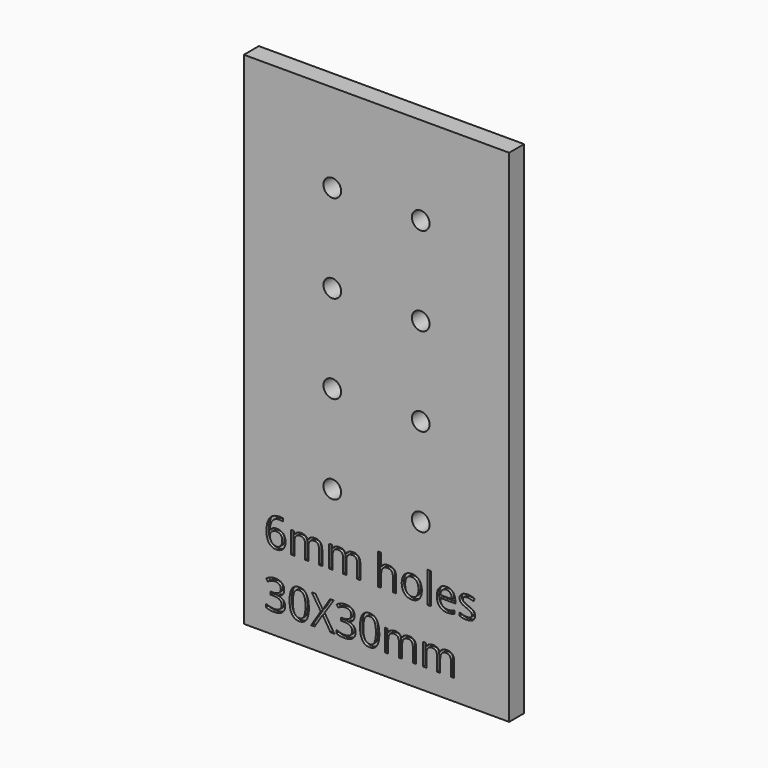
from build123d import *

# Parameters (mm, degrees)
F0_W         = 90
F0_H         = 170
F0_R         = 3
F1_DEPTH     = 6.35
F0_R_2       = 1.5
F3_TEXT_SIZE = 13.8888888889
F4_DEPTH     = 1


# Not quite as in the source:
# - Text() gives the source's letters only with a copy of the font that has no kerning and outlines rounded to 1/6400 em; it was checked with that copy


with BuildPart() as f1:
    # F0 (on Front) → F1 (new body)
    with BuildSketch(Plane.XZ):
        Rectangle(F0_W, F0_H)
        with Locations((-15, -35)):
            Circle(F0_R, mode=Mode.SUBTRACT)
        with Locations((-15, -5)):
            Circle(F0_R, mode=Mode.SUBTRACT)
        with Locations((15, -35)):
            Circle(F0_R, mode=Mode.SUBTRACT)
        with Locations((15, -5)):
            Circle(F0_R, mode=Mode.SUBTRACT)
        with Locations((-15, 25)):
            Circle(F0_R, mode=Mode.SUBTRACT)
        with Locations((15, 25)):
            Circle(F0_R, mode=Mode.SUBTRACT)
        with Locations((-15, 55)):
            Circle(F0_R, mode=Mode.SUBTRACT)
        with Locations((15, 55)):
            Circle(F0_R, mode=Mode.SUBTRACT)
    extrude(amount=F1_DEPTH)

    # F3 (on face) → F4 (cut)
    with BuildSketch(Plane.XZ.offset(6.35)):
        with Locations((-38.13868023, -59.0854487956)):
            Text('6mm holes', F3_TEXT_SIZE, font='Open Sans', text_align=(TextAlign.LEFT, TextAlign.BOTTOM))
        with Locations((-38.13868023, -77.9743376845)):
            Text('30X30mm', F3_TEXT_SIZE, font='Open Sans', text_align=(TextAlign.LEFT, TextAlign.BOTTOM))
    extrude(amount=-F4_DEPTH, mode=Mode.SUBTRACT)


with BuildPart() as f1b:
    # F0 (on Front) → F1, piece 2 (new body)
    with BuildSketch(Plane.XZ):
        with Locations((-415, 250)):
            Circle(F0_R_2)
    extrude(amount=F1_DEPTH)


solid = f1.part
